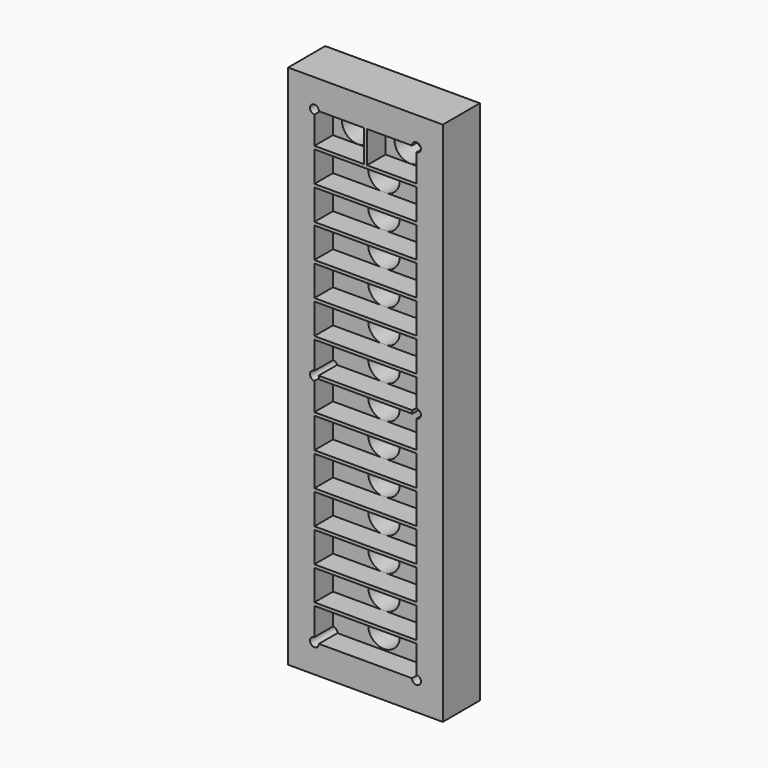
from build123d import *

# Parameters (mm, degrees)
F0_W      = 63.5
F0_H      = 215.9
F1_DEPTH  = 19.05
F2_W      = 41.91
F2_H      = 192.532
F3_DEPTH  = 9.525
F5_D      = 3.6576
F5_DEPTH  = 19.05
F5_START  = 9.525
F5_TIP    = 1.0988539001
F6_R      = 1.8288
F7_DEPTH  = 5.08
F8_W      = 41.91
F8_H      = 1.27
F9_DEPTH  = 9.525
F10_W     = 0.635
F10_H     = 13.1172857143
F11_DEPTH = 9.525
F12_R     = 6.5
F13_DEPTH = 25.4
F14_R     = 6.5
F15_DEPTH = 25.4
F16_R     = 6.5
F17_DEPTH = 25.4


# Not quite as in the source:
# - after a boolean that leaves OpenCascade's solid faulty, fix() repairs it


with BuildPart() as f1:
    # F0 (on Front) → F1 (new body)
    with BuildSketch(Plane.XZ):
        Rectangle(F0_W, F0_H)
    extrude(amount=F1_DEPTH)

    # F2 (on face) → F3 (cut)
    with BuildSketch(Plane.XZ.offset(19.05)):
        Rectangle(F2_W, F2_H)
    extrude(amount=-F3_DEPTH, mode=Mode.SUBTRACT)

    # F5
    # its depths count from where the whole tool has entered the part; down to there all is cleared
    with Locations(Plane.XZ.offset(19.05).offset(-F5_START)):
        with Locations((-20.955, -96.266), (-20.955, 0), (20.955, 0), (20.955, -96.266), (-20.955, 96.266), (20.955, 96.266)):
            Hole(F5_D / 2, depth=F5_DEPTH)
            with Locations((0, 0, -(F5_DEPTH + F5_TIP / 2))):  # 118° drill point
                Cone(0, F5_D / 2, F5_TIP, mode=Mode.SUBTRACT)

    # F6 (on face) → F7 (cut)
    with BuildSketch(Plane(origin=(0, 0, 0), x_dir=(-1, 0, 0), z_dir=(0, 1, 0))):
        Polygon((-16.262297012, 96.266), (-18.608648506, 100.33), (-23.301351494, 100.33), (-25.647702988, 96.266), (-23.301351494, 92.202), (-18.608648506, 92.202), align=None)
        with Locations((-20.955, 96.266)):
            Circle(F6_R, mode=Mode.SUBTRACT)
        Polygon((23.301351494, 92.202), (25.647702988, 96.266), (23.301351494, 100.33), (18.608648506, 100.33), (16.262297012, 96.266), (18.608648506, 92.202), align=None)
        with Locations((20.955, 96.266)):
            Circle(F6_R, mode=Mode.SUBTRACT)
        Polygon((-18.608648506, -4.064), (-16.262297012, 0), (-18.608648506, 4.064), (-23.301351494, 4.064), (-25.647702988, 0), (-23.301351494, -4.064), align=None)
        with Locations((-20.955, 0)):
            Circle(F6_R, mode=Mode.SUBTRACT)
        Polygon((23.301351494, -4.064), (25.647702988, 0), (23.301351494, 4.064), (18.608648506, 4.064), (16.262297012, 0), (18.608648506, -4.064), align=None)
        with Locations((20.955, 0)):
            Circle(F6_R, mode=Mode.SUBTRACT)
        Polygon((-18.608648506, -100.33), (-16.262297012, -96.266), (-18.608648506, -92.202), (-23.301351494, -92.202), (-25.647702988, -96.266), (-23.301351494, -100.33), align=None)
        with Locations((-20.955, -96.266)):
            Circle(F6_R, mode=Mode.SUBTRACT)
        Polygon((23.301351494, -100.33), (25.647702988, -96.266), (23.301351494, -92.202), (18.608648506, -92.202), (16.262297012, -96.266), (18.608648506, -100.33), align=None)
        with Locations((20.955, -96.266)):
            Circle(F6_R, mode=Mode.SUBTRACT)
    extrude(amount=-F7_DEPTH, mode=Mode.SUBTRACT)

    # F8 (on face) → F9 (join, through all)
    with BuildSketch(Plane.XZ.offset(9.525)):
        with BuildLine():
            ThreePointArc((19.1262, 0), (19.154870403, 0.3225567765), (19.2399826706, 0.635))
            Line((19.2399826706, 0.635), (-19.2399826706, 0.635))
            ThreePointArc((-19.2399826706, 0.635), (-19.154870403, 0.3225567765), (-19.1262, 0))
            ThreePointArc((-19.1262, 0), (-19.154870403, -0.3225567765), (-19.2399826706, -0.635))
            Line((-19.2399826706, -0.635), (19.2399826706, -0.635))
            ThreePointArc((19.2399826706, -0.635), (19.154870403, -0.3225567765), (19.1262, 0))
        make_face()
        with Locations((0, 13.7522857143)):
            Rectangle(F8_W, F8_H)
        with Locations((0, -13.7522857143)):
            Rectangle(F8_W, F8_H)
        with Locations((0, 27.5045714286)):
            Rectangle(F8_W, F8_H)
        with Locations((0, -27.5045714286)):
            Rectangle(F8_W, F8_H)
        with Locations((0, 41.2568571429)):
            Rectangle(F8_W, F8_H)
        with Locations((0, -41.2568571429)):
            Rectangle(F8_W, F8_H)
        with Locations((0, 55.0091428571)):
            Rectangle(F8_W, F8_H)
        with Locations((0, -55.0091428571)):
            Rectangle(F8_W, F8_H)
        with Locations((0, 68.7614285714)):
            Rectangle(F8_W, F8_H)
        with Locations((0, -68.7614285714)):
            Rectangle(F8_W, F8_H)
        with Locations((0, 82.5137142857)):
            Rectangle(F8_W, F8_H)
        with Locations((0, -82.5137142857)):
            Rectangle(F8_W, F8_H)
    extrude(amount=F9_DEPTH)

    add(f1.part.fix(), mode=Mode.REPLACE)

    # F10 (on face) → F11 (join, through all)
    with BuildSketch(Plane.XZ.offset(9.525)):
        with Locations((-0.3175, 89.7073571429)):
            Rectangle(F10_W, F10_H)
        with Locations((0.3175, 89.7073571429)):
            Rectangle(F10_W, F10_H)
    extrude(amount=F11_DEPTH)

    # F12 (on face) → F13 (cut)
    with BuildSketch(Plane.XZ.offset(9.525)):
        with Locations((-10.795, 89.7073571429)):
            Circle(F12_R)
    extrude(amount=-F13_DEPTH, mode=Mode.SUBTRACT)

    # F14 (on face) → F15 (cut)
    with BuildSketch(Plane.XZ.offset(9.525)):
        with Locations((10.795, 89.7073571429)):
            Circle(F14_R)
    extrude(amount=-F15_DEPTH, mode=Mode.SUBTRACT)

    # F16 (on face) → F17 (cut)
    with BuildSketch(Plane.XZ.offset(9.525)):
        with Locations((0, 75.6375714286)):
            Circle(F16_R)
        with Locations((0, 61.8961714286)):
            Circle(F16_R)
        with Locations((0, 48.1547714286)):
            Circle(F16_R)
        with Locations((0, 34.4133714286)):
            Circle(F16_R)
        with Locations((0, 20.6719714286)):
            Circle(F16_R)
        with Locations((0, 6.9305714286)):
            Circle(F16_R)
        with Locations((0, -6.8108285714)):
            Circle(F16_R)
        with Locations((0, -20.5522285714)):
            Circle(F16_R)
        with Locations((0, -34.2936285714)):
            Circle(F16_R)
        with Locations((0, -48.0350285714)):
            Circle(F16_R)
        with Locations((0, -61.7764285714)):
            Circle(F16_R)
        with Locations((0, -75.5178285714)):
            Circle(F16_R)
        with Locations((0, -89.2592285714)):
            Circle(F16_R)
    extrude(amount=-F17_DEPTH, mode=Mode.SUBTRACT)


solid = f1.part
